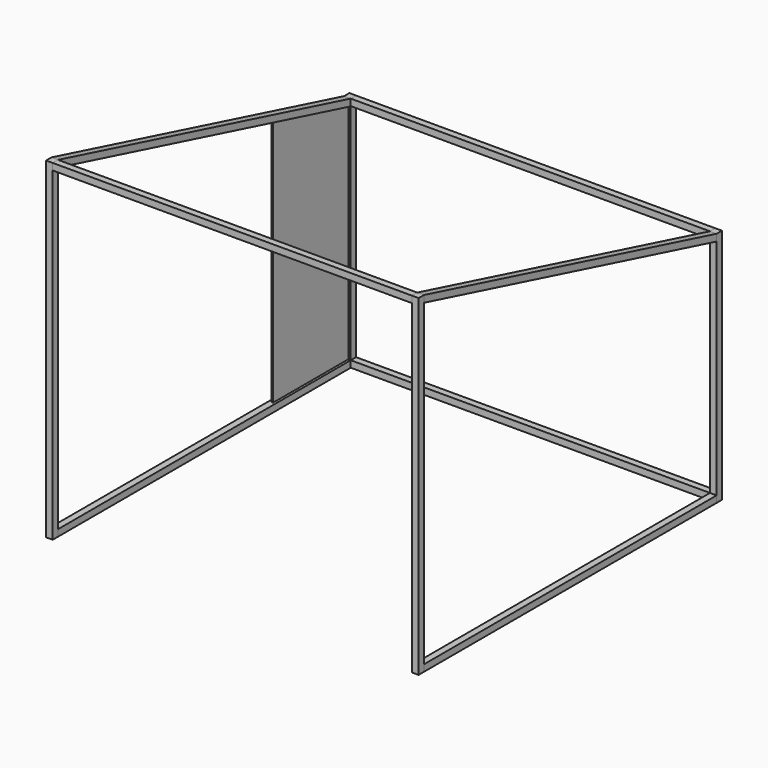
from build123d import *

# Parameters (mm, degrees)
F2_W          = 70
F2_H          = 3500
F3_DEPTH      = 70
F4_W          = 3790
F4_H          = 70
F5_DEPTH      = 70
F9_DEPTH      = 35
F9_DEPTH_BACK = 35
F8_W          = 3860
F8_H          = 70
F11_W         = 70
F11_H         = 2500
F12_DEPTH     = 70
F11_W_2       = 3789.998
F11_H_2       = 70
F14_DEPTH     = 9


with BuildPart() as f3:
    # F2 (on Front) → F3 (new body)
    with BuildSketch(Plane.XZ):
        with Locations((-1930, 0)):
            Rectangle(F2_W, F2_H)
    extrude(amount=F3_DEPTH)


with BuildPart() as f3b:
    # F2 (on Front) → F3, piece 2 (new body)
    with BuildSketch(Plane.XZ):
        with Locations((1930, 0)):
            Rectangle(F2_W, F2_H)
    extrude(amount=F3_DEPTH)


with BuildPart() as f5:
    # F4 (on face) → F5 (new body)
    with BuildSketch(Plane.XZ):
        with Locations((0, 1715)):
            Rectangle(F4_W, F4_H)
    extrude(amount=F5_DEPTH)


with BuildPart() as f9:
    # F8 (on offset) → F9 (new body, two sides)
    with BuildSketch(Plane(origin=(-1930, 0, 0), x_dir=(0, -1, 0), z_dir=(-1, 0, 0))) as f9_sk:
        Polygon((0, 1677.6890887274), (0, 1750), (-3860, 750), (-3860, 677.6890887274), align=None)
    extrude(amount=F9_DEPTH)
    extrude(f9_sk.sketch, amount=-F9_DEPTH_BACK)


with BuildPart() as f9b:
    # F8 (on offset) → F9, piece 2 (new body, two sides)
    with BuildSketch(Plane(origin=(-1930, 0, 0), x_dir=(0, -1, 0), z_dir=(-1, 0, 0))) as f9_2_sk:
        with Locations((-1930, -1715)):
            Rectangle(F8_W, F8_H)
    extrude(amount=F9_DEPTH)
    extrude(f9_2_sk.sketch, amount=-F9_DEPTH_BACK)


with BuildPart() as f10_1:
    # F10: instance of F9
    add(f9.part.mirror(Plane.YZ))


with BuildPart() as f10_2:
    # F10: instance of F9b
    add(f9b.part.mirror(Plane.YZ))


with BuildPart() as f12:
    # F11 (on face) → F12 (new body)
    with BuildSketch(Plane(origin=(0, 3860, 0), x_dir=(-1, 0, 0), z_dir=(0, 1, 0))):
        with Locations((-1930, -500)):
            Rectangle(F11_W, F11_H)
    extrude(amount=F12_DEPTH)


with BuildPart() as f12b:
    # F11 (on face) → F12, piece 2 (new body)
    with BuildSketch(Plane(origin=(0, 3860, 0), x_dir=(-1, 0, 0), z_dir=(0, 1, 0))):
        with Locations((1930, -500)):
            Rectangle(F11_W, F11_H)
    extrude(amount=F12_DEPTH)


with BuildPart() as f12c:
    # F11 (on face) → F12, piece 3 (new body)
    with BuildSketch(Plane(origin=(0, 3860, 0), x_dir=(-1, 0, 0), z_dir=(0, 1, 0))):
        with Locations((0, 715)):
            Rectangle(F11_W_2, F11_H_2)
    extrude(amount=F12_DEPTH)


with BuildPart() as f12d:
    # F11 (on face) → F12, piece 4 (new body)
    with BuildSketch(Plane(origin=(0, 3860, 0), x_dir=(-1, 0, 0), z_dir=(0, 1, 0))):
        with Locations((0, -1715)):
            Rectangle(F11_W_2, F11_H_2)
    extrude(amount=F12_DEPTH)


with BuildPart() as f14:
    # F13 (on offset) → F14 (new body, symmetric)
    with BuildSketch(Plane(origin=(-1930, 0, 0), x_dir=(0, -1, 0), z_dir=(-1, 0, 0))):
        Polygon((-2870, 944.495902847), (-3870, 685.4285453341), (-3870, -1690), (-2870, -1690), align=None)
    extrude(amount=F14_DEPTH, both=True)


solid = Compound([f3.part, f3b.part, f5.part, f9.part, f9b.part, f10_1.part, f10_2.part, f12.part, f12b.part, f12c.part, f12d.part, f14.part])
